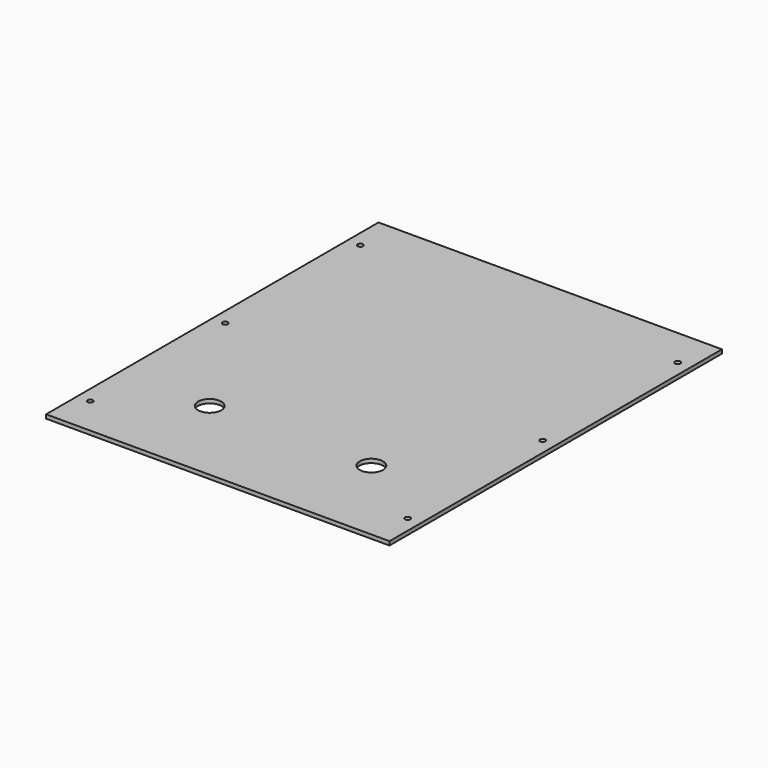
from build123d import *

# Parameters (mm, degrees)
F1_W     = 264.5
F1_H     = 320
F2_DEPTH = 3
F4_D     = 4.2
F4_DEPTH = 4
F4_TIP   = 1.2618073
F5_R     = 9
F6_DEPTH = 3


# Not quite as in the source:
# - a pattern or mirror of a feature is missing from the dataset's text; its kind, count and spacing are read off the source's solid


with BuildPart() as f2:
    # F1 (on Top) → F2 (new body)
    with BuildSketch(Plane.XY):
        Rectangle(F1_W, F1_H)
    extrude(amount=F2_DEPTH)

    # F4
    with Locations(Plane.XY.offset(3)):
        with Locations((-122.25, 130), (-122.25, 0), (-122.25, -130)):
            f4 = Hole(F4_D / 2, depth=F4_DEPTH)
            with Locations((0, 0, -(F4_DEPTH + F4_TIP / 2))):  # 118° drill point
                Cone(0, F4_D / 2, F4_TIP, mode=Mode.SUBTRACT)

    # F4_copies: F4 across plane
    add(f4.mirror(Plane(origin=(0, 0, 0), x_dir=(0, 0, 1), z_dir=(1, 0, 0))), mode=Mode.SUBTRACT)

    # F5 (on face) → F6 (cut, through all)
    with BuildSketch(Plane.XY.offset(3)):
        with Locations((-62.25, -90)):
            Circle(F5_R)
        with Locations((62.25, -90)):
            Circle(F5_R)
    extrude(amount=-F6_DEPTH, mode=Mode.SUBTRACT)


solid = f2.part
